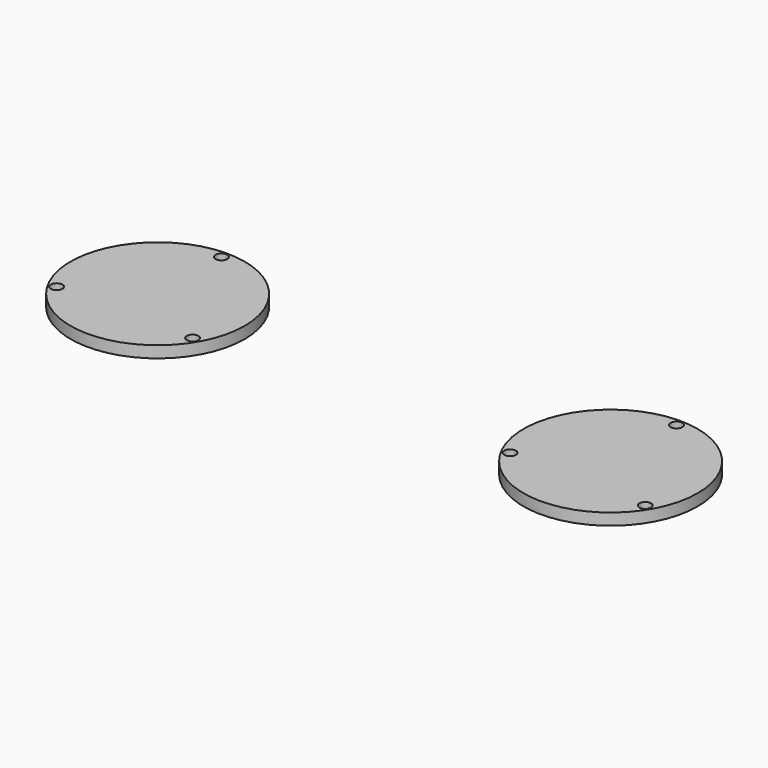
from build123d import *

# Parameters (mm, degrees)
F0_R     = 11.9
F0_R_2   = 0.8
F1_DEPTH = 1.5875
F2_R     = 11.9
F2_R_2   = 0.8
F3_DEPTH = 1.5875


# Not quite as in the source:
# - a length typed as a fraction of an inch, garbled in the dataset ("3 / 203.2 mm" for 3/8 in), is restored


with BuildPart() as f1:
    # F0 (on Top) → F1 (new body)
    with BuildSketch(Plane.XY):
        Circle(F0_R)
        with Locations((-9.4334447669, -5.4607801485)):
            Circle(F0_R_2, mode=Mode.SUBTRACT)
        with Locations((9.3155007377, -5.6596330275)):
            Circle(F0_R_2, mode=Mode.SUBTRACT)
        with Locations((0, 10.9)):
            Circle(F0_R_2, mode=Mode.SUBTRACT)
    extrude(amount=F1_DEPTH)


with BuildPart() as f3:
    # F2 (on Top) → F3 (new body)
    with BuildSketch(Plane.XY):
        with Locations((61.8878431498, 0)):
            Circle(F2_R)
        with Locations((52.3094763812, -5.2023927231)):
            Circle(F2_R_2, mode=Mode.SUBTRACT)
        with Locations((71.1824307928, -5.6939125869)):
            Circle(F2_R_2, mode=Mode.SUBTRACT)
        with Locations((62.1716222755, 10.89630531)):
            Circle(F2_R_2, mode=Mode.SUBTRACT)
    extrude(amount=F3_DEPTH)


solid = Compound([f1.part, f3.part])
